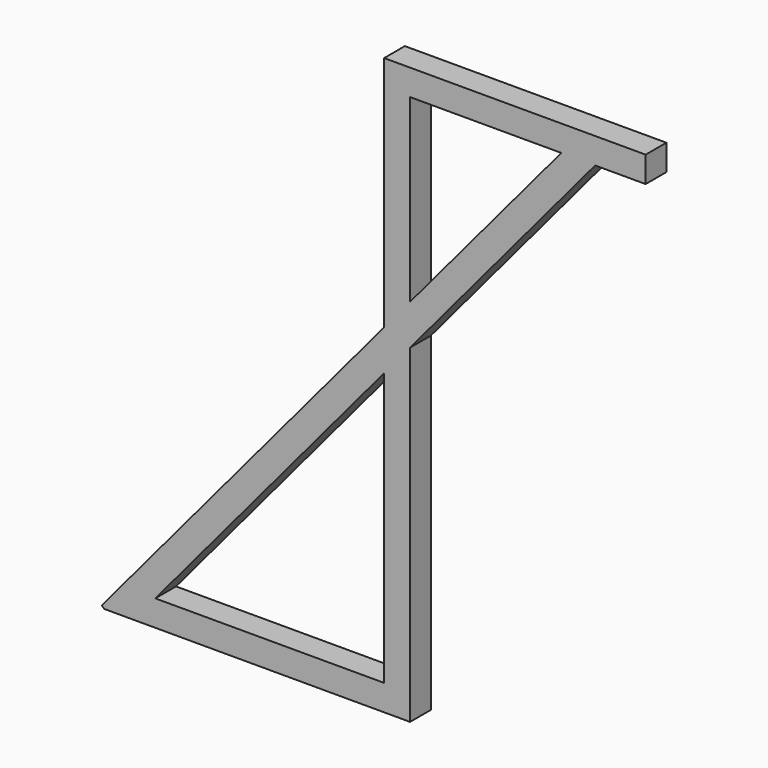
from build123d import *

# Parameters (mm, degrees)
F0_W     = 45
F0_H     = 45
F1_DEPTH = 45


with BuildPart() as f1:
    # F0 (on Front) → F1 (new body)
    with BuildSketch(Plane.XZ):
        Polygon((139.1122582526, 518.4320460093), (139.1122582526, 588.439618218), (-316.8877249613, 45), (-258.1443969413, 45), align=None)
        Polygon((-258.1443969413, 45), (-316.8877249613, 45), (-351.3597249985, 3.9178701118), (-346.6905892175, 0), (-295.9038803443, 0), align=None)
        Polygon((139.1122582526, 0), (139.1122582526, 45), (-258.1443969413, 45), (-295.9038803443, 0), align=None)
        with Locations((161.6122582526, 22.5)):
            Rectangle(F0_W, F0_H)
        Polygon((184.1122582526, 45), (184.1122582526, 572.060957676), (139.1122582526, 518.4320460093), (139.1122582526, 45), align=None)
        Polygon((184.1122582526, 600), (148.8125703421, 600), (139.1122582526, 588.439618218), (139.1122582526, 518.4320460093), (184.1122582526, 572.060957676), align=None)
        Polygon((184.1122582526, 642.0685298847), (184.1122582526, 600), (184.1122582526, 572.060957676), (505.43626743, 955), (446.6929394101, 955), align=None)
        with Locations((161.6122582526, 977.5)):
            Rectangle(F0_W, F0_H)
        Polygon((184.1122582526, 1000), (184.1122582526, 955), (446.6929394101, 955), (484.264167594, 999.7756461664), (518.7361675344, 970.8502037305), (505.43626743, 955), (593.1122582526, 955), (593.1122582526, 1000), align=None)
        Polygon((139.1122582526, 588.439618218), (148.8125703421, 600), (184.1122582526, 642.0685298847), (184.1122582526, 955), (139.1122582526, 955), align=None)
        Polygon((484.264167594, 999.7756461664), (446.6929394101, 955), (505.43626743, 955), (518.7361675344, 970.8502037305), align=None)
        Polygon((184.1122582526, 642.0685298847), (148.8125703421, 600), (184.1122582526, 600), align=None)
    extrude(amount=F1_DEPTH)


solid = f1.part
